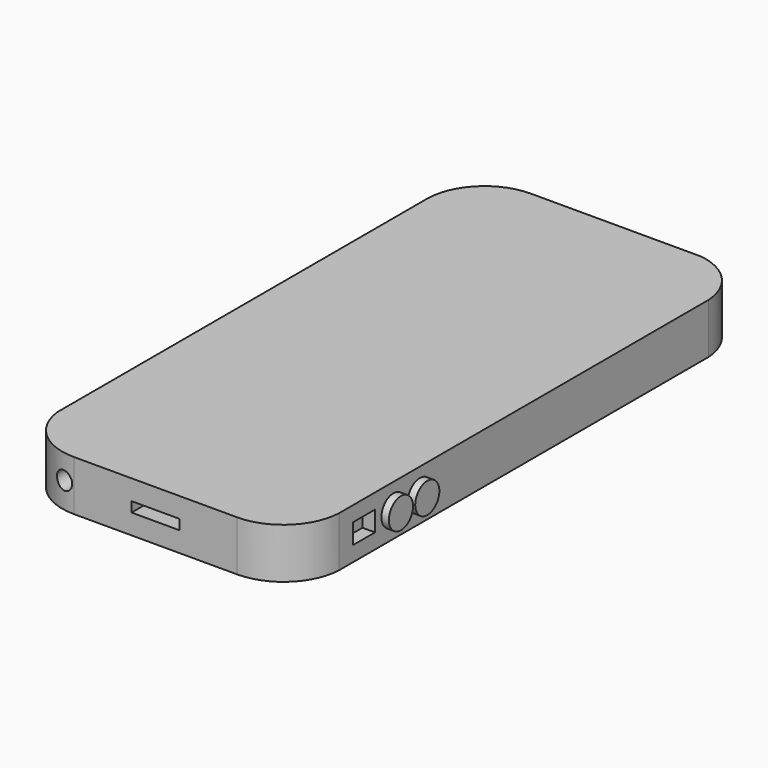
from build123d import *

# Parameters (mm, degrees)
F0_W      = 140.7454609871
F0_H      = 288.360491395
F1_DEPTH  = 25.4
F4_DEPTH  = 25.4
F6_W      = 16.9358227252
F6_H      = 4.5118425041
F7_DEPTH  = 3.81
F8_W      = 13.9597124967
F8_H      = 10.16
F9_DEPTH  = 6.35
F8_R      = 7.62
F11_DEPTH = 3.81
F5_W      = 24.153170515
F5_H      = 5.08
F12_DEPTH = 25.4
F5_R      = 4.5118428767
F13_DEPTH = 25.4


with BuildPart() as f1:
    # F0 (on Top) → F1 (new body)
    with BuildSketch(Plane.XY):
        with Locations((-3.7190392613, -27.8867259622)):
            Rectangle(F0_W, F0_H)
    extrude(amount=F1_DEPTH)

    # F2 (on face) → F4 (cut)
    with BuildSketch(Plane.XY.offset(25.4)):
        with BuildLine():
            ThreePointArc((66.6536912322, -144.3410718666), (57.604458326, -164.0297686766), (37.4814176394, -172.0669716597))
            Line((37.4814176394, -172.0669716597), (66.6536912322, -172.0669716597))
            Line((66.6536912322, -172.0669716597), (66.6536912322, -144.3410718666))
        make_face()
        with BuildLine():
            Line((-74.0917697549, -172.0669716597), (-45.0917528756, -172.0669716597))
            ThreePointArc((-45.0917528756, -172.0669716597), (-64.4708824202, -164.7127131958), (-74.0917697549, -146.3531296941))
            Line((-74.0917697549, -146.3531296941), (-74.0917697549, -172.0669716597))
        make_face()
        with BuildLine():
            ThreePointArc((41.1493752002, 116.2935197353), (58.7544153268, 107.3576281035), (66.6536912322, 89.2637330754))
            Line((66.6536912322, 89.2637330754), (66.6536912322, 116.2935197353))
            Line((66.6536912322, 116.2935197353), (41.1493752002, 116.2935197353))
        make_face()
        with BuildLine():
            Line((-74.0917697549, 116.2935197353), (-74.0917697549, 87.8933618236))
            ThreePointArc((-74.0917697549, 87.8933618236), (-65.2592523832, 108.0224737135), (-44.8929982774, 116.2935197353))
            Line((-44.8929982774, 116.2935197353), (-74.0917697549, 116.2935197353))
        make_face()
    extrude(amount=-F4_DEPTH, mode=Mode.SUBTRACT)

    # F6 (on face) → F7 (join)
    with BuildSketch(Plane(origin=(0, 116.2935197353, 0), x_dir=(-1, 0, 0), z_dir=(0, 1, 0))):
        with Locations((-32.6814638376, 13.2347373292)):
            Rectangle(F6_W, F6_H)
    extrude(amount=F7_DEPTH)

    # F8 (on face) → F9 (cut)
    with BuildSketch(Plane.YZ.offset(66.6536912322)):
        with Locations((-128.4659260378, 12.7)):
            Rectangle(F8_W, F8_H)
    extrude(amount=-F9_DEPTH, mode=Mode.SUBTRACT)

    # F8 (on face) → F11 (join)
    with BuildSketch(Plane.YZ.offset(66.6536912322)):
        with Locations((-109.8529842751, 12.7)):
            Circle(F8_R)
        with Locations((-93.2342812741, 12.7)):
            Circle(F8_R)
    extrude(amount=F11_DEPTH)

    # F5 (on face) → F12 (cut)
    with BuildSketch(Plane.XZ.offset(172.0669716597)):
        with Locations((-3.8051676181, 12.7)):
            Rectangle(F5_W, F5_H)
    extrude(amount=-F12_DEPTH, mode=Mode.SUBTRACT)

    # F5 (on face) → F13 (cut)
    with BuildSketch(Plane.XZ.offset(172.0669716597)):
        with Locations((-50.3822378814, 13.0843427032)):
            Circle(F5_R)
    extrude(amount=-F13_DEPTH, mode=Mode.SUBTRACT)


solid = f1.part
